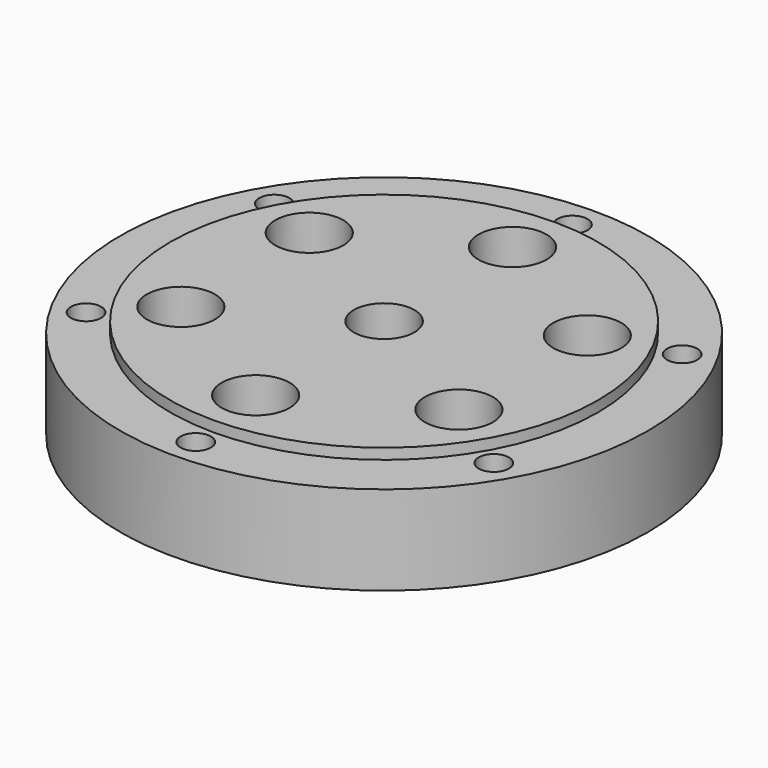
from build123d import *

# Parameters (mm, degrees)
F0_R            = 74
F1_DEPTH        = 25
F2_R            = 60
F3_DEPTH        = 3
F4_D            = 17
F6_D            = 8.5
F6_COPIES_COUNT = 6
F8_D            = 12.7
F8_CBORE_D      = 19.1
F8_CBORE_DEPTH  = 13.1
F8_COPIES_COUNT = 6


# Not quite as in the source:
# - a pattern or mirror of a feature is missing from the dataset's text; its kind, count and spacing are read off the source's solid


with BuildPart() as f1:
    # F0 (on Top) → F1 (new body)
    with BuildSketch(Plane.XY):
        Circle(F0_R)
    extrude(amount=F1_DEPTH)

    # F2 (on face) → F3 (join)
    with BuildSketch(Plane.XY.offset(25)):
        Circle(F2_R)
    extrude(amount=F3_DEPTH)

    # F4 (through all)
    with Locations(Plane(origin=(0, 0, 0), x_dir=(1, 0, 0), z_dir=(0, 0, -1))):
        with Locations((0, 0)):
            Hole(F4_D / 2)

    # F6 (through all)
    with Locations(Plane.XY.offset(25)):
        with Locations((0, 66)):
            f6 = Hole(F6_D / 2)

    # F6_copies: F6 ×6 about axis
    f6_copies_axis = Axis((0, 0, 0), (0, 0, 1))
    for i in range(1, F6_COPIES_COUNT):
        add(f6.rotate(f6_copies_axis, i * 360 / F6_COPIES_COUNT), mode=Mode.SUBTRACT)

    # F8 (through all)
    with Locations(Plane.XY.offset(28)):
        with Locations((0, 45)):
            f8 = CounterBoreHole(F8_D / 2, F8_CBORE_D / 2, F8_CBORE_DEPTH)

    # F8_copies: F8 ×6 about axis
    f8_copies_axis = Axis((0, 0, 0), (0, 0, 1))
    for i in range(1, F8_COPIES_COUNT):
        add(f8.rotate(f8_copies_axis, i * 360 / F8_COPIES_COUNT), mode=Mode.SUBTRACT)


solid = f1.part
